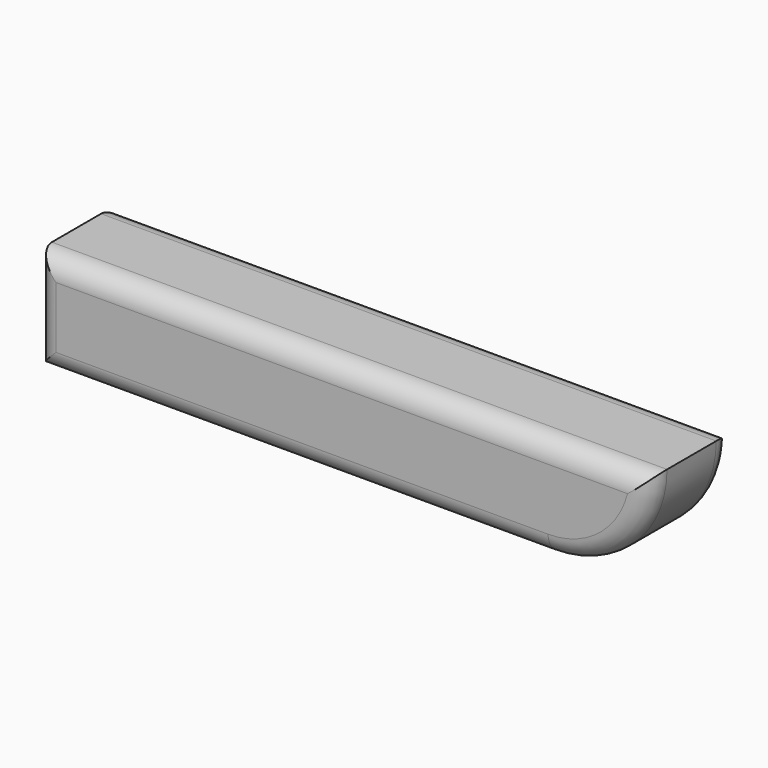
from build123d import *

# Parameters (mm, degrees)
F0_W     = 127
F0_H     = 25.4
F1_DEPTH = 25.4
F2_R     = 5.08


# Not quite as in the source:
# - a feature names something its author has since deleted; it is built from what else it names


with BuildPart() as f1:
    # F0 (on Front) → F1 (new body)
    with BuildSketch(Plane.XZ):
        with Locations((-12.2346525788, -22.7242771864)):
            Rectangle(F0_W, F0_H)
        with BuildLine():
            Line((76.6653474212, -10.0242771864), (51.2653474212, -10.0242771864))
            Line((51.2653474212, -10.0242771864), (51.2653474212, -35.4242771864))
            ThreePointArc((51.2653474212, -35.4242771864), (69.2258596633, -27.9847894285), (76.6653474212, -10.0242771864))
        make_face()
    extrude(amount=F1_DEPTH)

    # F2
    f2_edges = [f1.edges().sort_by_distance(p)[0] for p in [
        (-75.734653, -25.4, -22.724277),
        (-12.234653, -25.4, -35.424277),
        (69.22586, -25.4, -27.984789),
        (0.465347, -25.4, -10.024277),
        (-75.734653, 0, -22.724277),
        (-12.234653, 0, -35.424277),
        (69.22586, 0, -27.984789),
        (0.465347, 0, -10.024277),
    ]]
    fillet(f2_edges, radius=F2_R)


solid = f1.part
